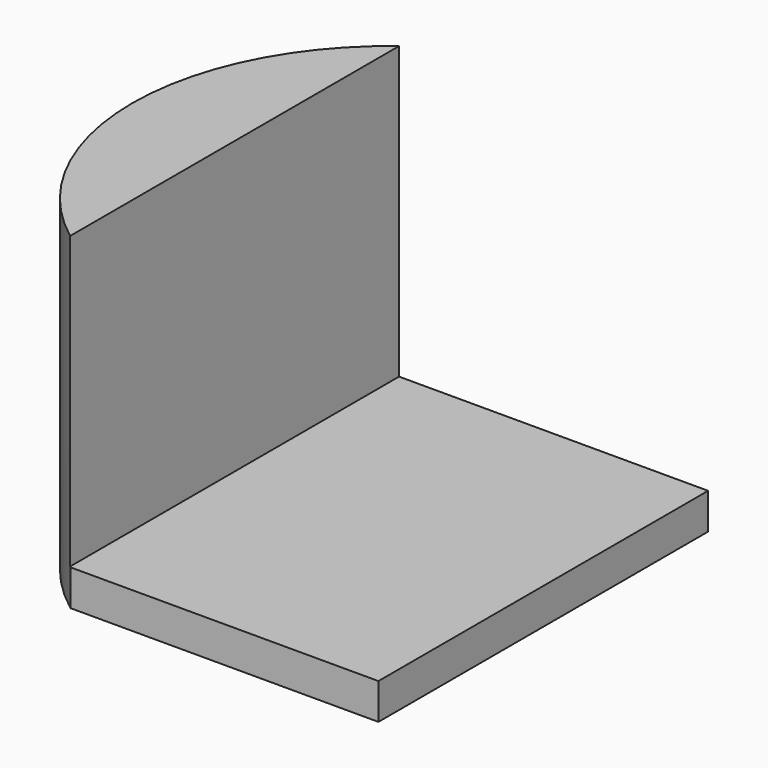
from build123d import *

# Parameters (mm, degrees)
F1_DEPTH = 2.794
F5_DEPTH = 25.4


# Not quite as in the source:
# - a feature of the source that left no trace in its solid (it failed there, or was rolled back) is left out
# - the program builds the solid bodies; features that only make, move or delete a surface that nothing else refers to are left out


with BuildPart() as f1:
    # F0 (on Top) → F1 (new body)
    with BuildSketch(Plane.XY):
        with BuildLine():
            Line((-16.4724217036, 22.0521983965), (-40.4838242176, 22.0521983965))
            Line((-40.4838242176, 22.0521983965), (-40.4838242176, -9.8933519139))
            ThreePointArc((-40.4838242176, -9.8933519139), (-40.4370025072, -9.928574703), (-40.3900778613, -9.963660242))
            Line((-40.3900778613, -9.963660242), (-16.4724217036, -9.963660242))
            Line((-16.4724217036, -9.963660242), (-16.4724217036, 22.0521983965))
        make_face()
    extrude(amount=F1_DEPTH)

    # F0 (on Top) → F5 (join)
    with BuildSketch(Plane.XY):
        with BuildLine():
            Line((-40.4838242176, -9.8933519139), (-40.4838242176, 22.0521983965))
            ThreePointArc((-40.4838242176, 22.0521983965), (-48.4410997737, 6.0794232413), (-40.4838242176, -9.8933519139))
        make_face()
    extrude(amount=F5_DEPTH)


solid = f1.part
